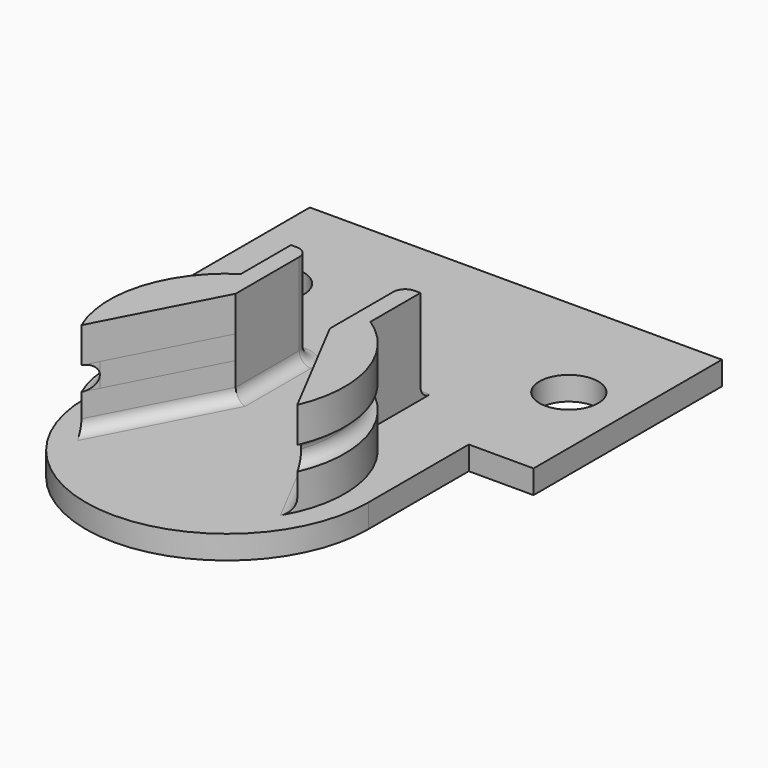
from build123d import *

# Parameters (mm, degrees)
F1_DEPTH     = 2
F3_DEPTH     = 3
F5_DEPTH     = 2
F7_DEPTH     = 3
F8_T4_ANGLE  = 102.3969146675
F8_T10_ANGLE = 102.3969146675
F8_T16_ANGLE = 102.3969146675
F8_T22_ANGLE = 102.3969146675
F8_T26_ANGLE = 121.7069479791
F8_T28_ANGLE = 121.7069479791
F8_T30_ANGLE = 121.7069479791
F8_T32_ANGLE = 121.7069479791
F9_W         = 24
F9_H         = 22.6653645039
F10_DEPTH    = 10
F11_R        = 2.5
F12_DEPTH    = 2
F13_R        = 1


# Not quite as in the source:
# - a fillet or chamfer that OpenCascade refuses, or shapes differently, is made with other operations: its cross-section is extruded or revolved along the edge and cut away or added


with BuildPart() as f1:
    # F0 (on Top) → F1 (new body)
    with BuildSketch(Plane.XY):
        with BuildLine():
            ThreePointArc((5.5, 1.5), (0, 24.1653645039), (-5.5, 1.5))
            Line((-5.5, 1.5), (-5.5, -1.5))
            ThreePointArc((-5.5, -1.5), (0, -24.1653645039), (5.5, -1.5))
            Line((5.5, -1.5), (5.5, 1.5))
        make_face()
    extrude(amount=F1_DEPTH)

    # F2 (on face) → F3 (join)
    with BuildSketch(Plane.XY.offset(2)):
        with BuildLine():
            Line((9.7844830762, 19.1125863177), (8.6602540378, 17.1653645039))
            ThreePointArc((8.6602540378, 17.1653645039), (9.4991255677, 9.0402063559), (4, 3.0002131139))
            Line((4, 3.0002131139), (4, -6.2432010007))
            Line((4, -6.2432010007), (9.1651513899, -16.1653645039))
            ThreePointArc((9.1651513899, -16.1653645039), (9.5868378212, -9.3206253964), (5.5, -3.8137179596))
            Line((5.5, -3.8137179596), (5.5, 1.5))
            ThreePointArc((5.5, 1.5), (11.6599594736, 9.3289327537), (9.7844830762, 19.1125863177))
        make_face()
        with BuildLine():
            ThreePointArc((-4, 3.0002131139), (-9.4991255677, 9.0402063559), (-8.6602540378, 17.1653645039))
            Line((-8.6602540378, 17.1653645039), (-9.7844830762, 19.1125863177))
            ThreePointArc((-9.7844830762, 19.1125863177), (-11.6599594736, 9.3289327537), (-5.5, 1.5))
            Line((-5.5, 1.5), (-5.5, -3.8137179596))
            ThreePointArc((-5.5, -3.8137179596), (-9.5868378212, -9.3206253964), (-9.1651513899, -16.1653645039))
            Line((-9.1651513899, -16.1653645039), (-4, -6.2432010007))
            Line((-4, -6.2432010007), (-4, 3.0002131139))
        make_face()
    extrude(amount=F3_DEPTH)

    # F4 (on face) → F5 (join)
    with BuildSketch(Plane.XY.offset(5)):
        with BuildLine():
            Line((-8.0717844057, 16.1461052023), (-9.7844830762, 19.1125863177))
            ThreePointArc((-9.7844830762, 19.1125863177), (-11.6599594736, 9.3289327537), (-5.5, 1.5))
            Line((-5.5, 1.5), (-5.5, -5.0414610795))
            ThreePointArc((-5.5, -5.0414610795), (-8.6043935433, -9.5263473097), (-8.5483759414, -14.980549891))
            Line((-8.5483759414, -14.980549891), (-4, -6.2432010007))
            Line((-4, -6.2432010007), (-4, 4.1031067556))
            ThreePointArc((-4, 4.1031067556), (-8.5258693153, 9.2827350759), (-8.0717844057, 16.1461052023))
        make_face()
        with BuildLine():
            ThreePointArc((5.5, 1.5), (11.6599594736, 9.3289327537), (9.7844830762, 19.1125863177))
            Line((9.7844830762, 19.1125863177), (8.0717844057, 16.1461052023))
            ThreePointArc((8.0717844057, 16.1461052023), (8.5258693153, 9.2827350759), (4, 4.1031067556))
            Line((4, 4.1031067556), (4, -6.2432010007))
            Line((4, -6.2432010007), (8.5483759414, -14.980549891))
            ThreePointArc((8.5483759414, -14.980549891), (8.6043935433, -9.5263473097), (5.5, -5.0414610795))
            Line((5.5, -5.0414610795), (5.5, 1.5))
        make_face()
    extrude(amount=F5_DEPTH)

    # F6 (on face) → F7 (join)
    with BuildSketch(Plane.XY.offset(7)):
        with BuildLine():
            Line((9.7844830762, 19.1125863177), (8.6602540378, 17.1653645039))
            ThreePointArc((8.6602540378, 17.1653645039), (9.4991255677, 9.0402063559), (4, 3.0002131139))
            Line((4, 3.0002131139), (4, -6.2432010007))
            Line((4, -6.2432010007), (9.1651513899, -16.1653645039))
            ThreePointArc((9.1651513899, -16.1653645039), (9.5868378212, -9.3206253964), (5.5, -3.8137179596))
            Line((5.5, -3.8137179596), (5.5, 1.5))
            ThreePointArc((5.5, 1.5), (11.6599594736, 9.3289327537), (9.7844830762, 19.1125863177))
        make_face()
        with BuildLine():
            ThreePointArc((-4, 3.0002131139), (-9.4991255677, 9.0402063559), (-8.6602540378, 17.1653645039))
            Line((-8.6602540378, 17.1653645039), (-9.7844830762, 19.1125863177))
            ThreePointArc((-9.7844830762, 19.1125863177), (-11.6599594736, 9.3289327537), (-5.5, 1.5))
            Line((-5.5, 1.5), (-5.5, -3.8137179596))
            ThreePointArc((-5.5, -3.8137179596), (-9.5868378212, -9.3206253964), (-9.1651513899, -16.1653645039))
            Line((-9.1651513899, -16.1653645039), (-4, -6.2432010007))
            Line((-4, -6.2432010007), (-4, 3.0002131139))
        make_face()
    extrude(amount=F7_DEPTH)

    # F8: fillet of radius 1 on 8 edges, made by hand


with BuildPart() as f8_tool2:
    # F8_s3 → F8_t4 (revolve)
    with BuildSketch(Plane(origin=(-4.1871135562, -1.6705281924, 0), x_dir=(0, 0, 1), z_dir=(0.9288065548, 0.3705649522, 0))):
        with BuildLine():
            ThreePointArc((6, 2.2992702923), (5.2928932188, 2.0063770734), (5, 1.2992702923))
            Line((5, 1.2992702923), (5, 2.2992702923))
            Line((5, 2.2992702923), (6, 2.2992702923))
        make_face()
    revolve(axis=Axis((0, -12.1653645039, 5), (0, 0, 1)), revolution_arc=F8_T4_ANGLE)

    split(bisect_by=Plane(origin=(-0.5900874414, 0.3071800789, 0), x_dir=(0, 0, 1), z_dir=(-0.8870108332, 0.4617486132, 0)), keep=Keep.TOP)

    split(bisect_by=Plane.YZ.offset(-4), keep=Keep.BOTTOM)


with BuildPart() as f1_1:
    add(f1.part)

    # F8_t1: union F8_tool2
    add(f8_tool2.part)


with BuildPart() as f8_tool8:
    # F8_s9 → F8_t10 (revolve)
    with BuildSketch(Plane(origin=(-4.1871135562, -1.6705281924, 0), x_dir=(0, 0, 1), z_dir=(0.9288065548, 0.3705649522, 0))):
        with BuildLine():
            ThreePointArc((7, 1.2992702923), (6.7071067812, 2.0063770734), (6, 2.2992702923))
            Line((6, 2.2992702923), (7, 2.2992702923))
            Line((7, 2.2992702923), (7, 1.2992702923))
        make_face()
    revolve(axis=Axis((0, -12.1653645039, 7), (0, 0, 1)), revolution_arc=F8_T10_ANGLE)

    split(bisect_by=Plane(origin=(-0.5900874414, 0.3071800789, 0), x_dir=(0, 0, 1), z_dir=(-0.8870108332, 0.4617486132, 0)), keep=Keep.TOP)

    split(bisect_by=Plane.YZ.offset(-4), keep=Keep.BOTTOM)


with BuildPart() as f1_2:
    add(f1_1.part)

    # F8_t7: union F8_tool8
    add(f8_tool8.part)


with BuildPart() as f8_tool14:
    # F8_s15 → F8_t16 (revolve)
    with BuildSketch(Plane(origin=(-5.6514123525, -8.3322514997, 0), x_dir=(0, 0, 1), z_dir=(-0.561323531, -0.8275964557, 0))):
        with BuildLine():
            ThreePointArc((6, -15.828705359), (6.7071067812, -16.1215985778), (7, -16.828705359))
            Line((7, -16.828705359), (7, -15.828705359))
            Line((7, -15.828705359), (6, -15.828705359))
        make_face()
    revolve(axis=Axis((0, -12.1653645039, 7), (0, 0, 1)), revolution_arc=F8_T16_ANGLE)

    split(bisect_by=Plane.YZ.offset(4), keep=Keep.TOP)

    split(bisect_by=Plane(origin=(0.5900874414, 0.3071800789, 0), x_dir=(0, 0, 1), z_dir=(0.8870108332, 0.4617486132, 0)), keep=Keep.TOP)


with BuildPart() as f1_3:
    add(f1_2.part)

    # F8_t13: union F8_tool14
    add(f8_tool14.part)


with BuildPart() as f8_tool20:
    # F8_s21 → F8_t22 (revolve)
    with BuildSketch(Plane(origin=(-5.6514123525, -8.3322514997, 0), x_dir=(0, 0, 1), z_dir=(-0.561323531, -0.8275964557, 0))):
        with BuildLine():
            ThreePointArc((5, -16.828705359), (5.2928932188, -16.1215985778), (6, -15.828705359))
            Line((6, -15.828705359), (5, -15.828705359))
            Line((5, -15.828705359), (5, -16.828705359))
        make_face()
    revolve(axis=Axis((0, -12.1653645039, 5), (0, 0, 1)), revolution_arc=F8_T22_ANGLE)

    split(bisect_by=Plane.YZ.offset(4), keep=Keep.TOP)

    split(bisect_by=Plane(origin=(0.5900874414, 0.3071800789, 0), x_dir=(0, 0, 1), z_dir=(0.8870108332, 0.4617486132, 0)), keep=Keep.TOP)


with BuildPart() as f1_4:
    add(f1_3.part)

    # F8_t19: union F8_tool20
    add(f8_tool20.part)

    # F8_s25 → F8_t26 (revolve, cut)
    with BuildSketch(Plane(origin=(-6.0530874143, 6.6819786169, 0), x_dir=(0, 0, 1), z_dir=(-0.6713698624, 0.7411224648, 0))):
        with BuildLine():
            ThreePointArc((7, 18.1674590926), (6.7071067812, 17.4603523114), (6, 17.1674590926))
            Line((6, 17.1674590926), (7, 17.1674590926))
            Line((7, 17.1674590926), (7, 18.1674590926))
        make_face()
    revolve(axis=Axis((0, 12.1653645039, 7), (0, 0, -1)), revolution_arc=F8_T26_ANGLE, mode=Mode.SUBTRACT)

    # F8_s27 → F8_t28 (revolve, cut)
    with BuildSketch(Plane(origin=(-2.1730837017, 0.4014208952, 0), x_dir=(0, 0, 1), z_dir=(0.9833630917, -0.1816508459, 0))):
        with BuildLine():
            ThreePointArc((6, -2.9629704506), (6.7071067812, -2.6700772318), (7, -1.9629704506))
            Line((7, -1.9629704506), (7, -2.9629704506))
            Line((7, -2.9629704506), (6, -2.9629704506))
        make_face()
    revolve(axis=Axis((0, 12.1653645039, 7), (0, 0, -1)), revolution_arc=F8_T28_ANGLE, mode=Mode.SUBTRACT)

    # F8_s29 → F8_t30 (revolve, cut)
    with BuildSketch(Plane(origin=(-2.1730837017, 0.4014208952, 0), x_dir=(0, 0, 1), z_dir=(0.9833630917, -0.1816508459, 0))):
        with BuildLine():
            ThreePointArc((5, -1.9629704506), (5.2928932188, -2.6700772318), (6, -2.9629704506))
            Line((6, -2.9629704506), (5, -2.9629704506))
            Line((5, -2.9629704506), (5, -1.9629704506))
        make_face()
    revolve(axis=Axis((0, 12.1653645039, 5), (0, 0, -1)), revolution_arc=F8_T30_ANGLE, mode=Mode.SUBTRACT)

    # F8_s31 → F8_t32 (revolve, cut)
    with BuildSketch(Plane(origin=(-6.0530874143, 6.6819786169, 0), x_dir=(0, 0, 1), z_dir=(-0.6713698624, 0.7411224648, 0))):
        with BuildLine():
            ThreePointArc((6, 17.1674590926), (5.2928932188, 17.4603523114), (5, 18.1674590926))
            Line((5, 18.1674590926), (5, 17.1674590926))
            Line((5, 17.1674590926), (6, 17.1674590926))
        make_face()
    revolve(axis=Axis((0, 12.1653645039, 5), (0, 0, -1)), revolution_arc=F8_T32_ANGLE, mode=Mode.SUBTRACT)

    # F9 (on face) → F10 (cut)
    with BuildSketch(Plane.XY.offset(10)):
        with Locations((0, 12.8326822519)):
            Rectangle(F9_W, F9_H)
    extrude(amount=-F10_DEPTH, mode=Mode.SUBTRACT)

    # F11 (on face) → F12 (join)
    with BuildSketch(Plane(origin=(0, 0, 0), x_dir=(1, 0, 0), z_dir=(0, 0, -1))):
        Polygon((12, 1.5), (12, 12.1653645039), (-12, 12.1653645039), (-12, 1.5), (-17.5, 1.5), (-17.5, -18.5), (17.5, -18.5), (17.5, 1.5), align=None)
        with Locations((-12.5, -8.5)):
            Circle(F11_R, mode=Mode.SUBTRACT)
        with Locations((12.5, -8.5)):
            Circle(F11_R, mode=Mode.SUBTRACT)
    extrude(amount=-F12_DEPTH)

    # F13
    f13_edges = [f1_4.edges().sort_by_distance(p)[0] for p in [
        (-4, 1.5, 6),
        (4, 1.5, 6),
        (4.75, 1.5, 2),
        (-4.75, 1.5, 2),
        (6.582576, -11.204283, 2),
        (-6.582576, -11.204283, 2),
        (-4, -2.371601, 2),
        (4, -2.371601, 2),
    ]]
    fillet(f13_edges, radius=F13_R)


solid = f1_4.part
